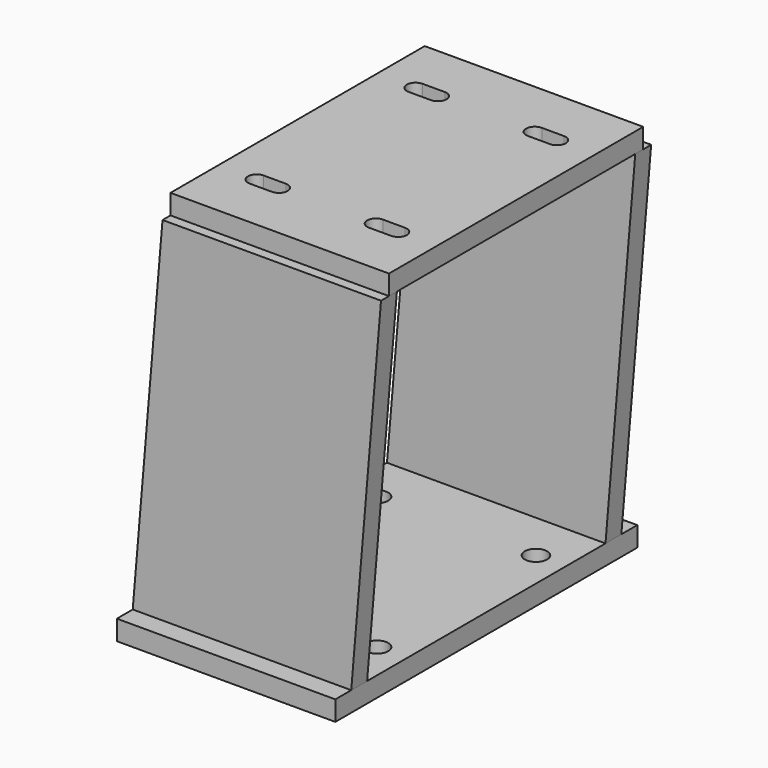
from build123d import *

# Parameters (mm, degrees)
F1_W      = 139.7
F1_H      = 241.3
F2_DEPTH  = 12.7
F4_D      = 14.2875
F5_W      = 139.7
F5_H      = 203.2
F6_DEPTH  = 12.7
F8_DEPTH  = 25.4
F10_DEPTH = 6.35


# Not quite as in the source:
# - a length typed as a fraction of an inch, garbled in the dataset ("3 / 203.2 mm" for 3/8 in), is restored


with BuildPart() as f2:
    # F1 (on Top) → F2 (new body)
    with BuildSketch(Plane.XY):
        Rectangle(F1_W, F1_H)
    extrude(amount=F2_DEPTH)

    # F4 (through all)
    with Locations(Plane.XY.offset(12.7)):
        with Locations((-50.8, 63.5), (50.8, 63.5), (50.8, -63.5), (-50.8, -63.5)):
            Hole(F4_D / 2)



with BuildPart() as f6:
    # F5 (on offset) → F6 (new body)
    with BuildSketch(Plane.XY.offset(250.825)):
        with Locations((19.05, 0)):
            Rectangle(F5_W, F5_H)
    extrude(amount=-F6_DEPTH)

    # F7 (on face) → F8 (cut)
    with BuildSketch(Plane.XY.offset(250.825)):
        with BuildLine():
            ThreePointArc((-26.162, -57.912), (-31.75, -63.5), (-26.162, -69.088))
            Line((-26.162, -69.088), (-11.938, -69.088))
            ThreePointArc((-11.938, -69.088), (-6.35, -63.5), (-11.938, -57.912))
            Line((-11.938, -57.912), (-26.162, -57.912))
        make_face()
        with BuildLine():
            Line((50.038, -69.088), (64.262, -69.088))
            ThreePointArc((64.262, -69.088), (69.85, -63.5), (64.262, -57.912))
            Line((64.262, -57.912), (50.038, -57.912))
            ThreePointArc((50.038, -57.912), (44.45, -63.5), (50.038, -69.088))
        make_face()
        with BuildLine():
            ThreePointArc((64.262, 57.912), (69.85, 63.5), (64.262, 69.088))
            Line((64.262, 69.088), (50.038, 69.088))
            ThreePointArc((50.038, 69.088), (44.45, 63.5), (50.038, 57.912))
            Line((50.038, 57.912), (64.262, 57.912))
        make_face()
        with BuildLine():
            Line((-11.938, 69.088), (-26.162, 69.088))
            ThreePointArc((-26.162, 69.088), (-31.75, 63.5), (-26.162, 57.912))
            Line((-26.162, 57.912), (-11.938, 57.912))
            ThreePointArc((-11.938, 57.912), (-6.35, 63.5), (-11.938, 69.088))
        make_face()
    extrude(amount=-F8_DEPTH, mode=Mode.SUBTRACT)


with BuildPart() as f2_1:
    add(f2.part)

    add(f6.part)  # F10 merges F6
    # F9 (on face) → F10 (join, symmetric)
    with BuildSketch(Plane.XZ.offset(101.6)):
        Polygon((88.9, 238.125), (-50.8, 238.125), (-69.85, 12.7), (69.85, 12.7), align=None)
    extrude(amount=F10_DEPTH, both=True)

    # F11: F2 across plane


with BuildPart() as f2_2:
    add(f2_1.part)
    add(f2_1.part.mirror(Plane.XZ))


solid = f2_2.part
